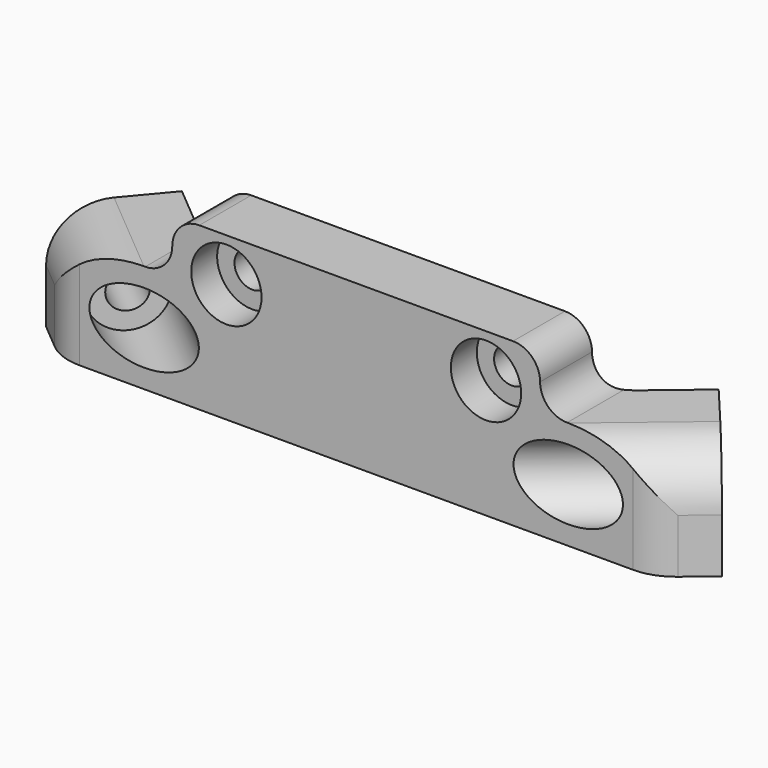
from build123d import *

# Parameters (mm, degrees)
F1_DEPTH       = 10
F2_W           = 34
F2_H           = 6
F3_DEPTH       = 5
F5_R           = 2.49999
F6_D           = 3.3
F6_CBORE_D     = 6.5
F6_CBORE_DEPTH = 3
F7_T1_DEPTH    = 28.1801488287
F7_T3_DEPTH    = 28.1801488287
F8_R           = 1.65
F9_DEPTH       = 49.9246466694
F10_R          = 1.65
F11_DEPTH      = 49.9246466694
F13_R          = 3.25
F14_DEPTH      = 25
F16_R          = 3.25
F17_DEPTH      = 25


# Not quite as in the source:
# - a fillet or chamfer that OpenCascade refuses, or shapes differently, is made with other operations: its cross-section is extruded or revolved along the edge and cut away or added
# - a fillet or chamfer is up to 0.001 mm smaller than in the source, because OpenCascade refuses the exact size


with BuildPart() as f1:
    # F0 (on Top) → F1 (new body)
    with BuildSketch(Plane.XY):
        with BuildLine():
            Line((-25.5868655417, 0), (0, 0))
            Line((0, 0), (25.5868655417, 0))
            ThreePointArc((25.5868655417, 0), (27.2969662583, 0.3015368961), (28.8008035901, 1.1697777844))
            Line((28.8008035901, 1.1697777844), (31.2369389286, 3.2139380484))
            Line((31.2369389286, 3.2139380484), (24.8090628318, 10.8743824796))
            Line((24.8090628318, 10.8743824796), (20.3940868771, 7.1697777844))
            ThreePointArc((20.3940868771, 7.1697777844), (18.8902495453, 6.3015368961), (17.1801488287, 6))
            Line((17.1801488287, 6), (0, 6))
            Line((0, 6), (-17.1801488287, 6))
            ThreePointArc((-17.1801488287, 6), (-18.8902495453, 6.3015368961), (-20.3940868771, 7.1697777844))
            Line((-20.3940868771, 7.1697777844), (-24.8090628318, 10.8743824796))
            Line((-24.8090628318, 10.8743824796), (-31.2369389286, 3.2139380484))
            Line((-31.2369389286, 3.2139380484), (-28.8008035901, 1.1697777844))
            ThreePointArc((-28.8008035901, 1.1697777844), (-27.2969662583, 0.3015368961), (-25.5868655417, 0))
        make_face()
    extrude(amount=F1_DEPTH)

    # F2 (on face) → F3 (join)
    with BuildSketch(Plane.XY.offset(10)):
        with Locations((0, 3)):
            Rectangle(F2_W, F2_H)
    extrude(amount=F3_DEPTH)

    # F5 (radius 2.5 in the source; OpenCascade refuses exactly that, so slightly less here)
    f5_edges = [f1.edges().sort_by_distance(p)[0] for p in [
        (17, 3, 10),
        (17, 3, 15),
        (-17, 3, 15),
        (-17, 3, 10),
    ]]
    fillet(f5_edges, radius=F5_R)

    # F6 (through all)
    with Locations(Plane.XZ):
        with Locations((-12, 11), (12, 11)):
            CounterBoreHole(F6_D / 2, F6_CBORE_D / 2, F6_CBORE_DEPTH)

    # F7: fillet of radius 5 on 2 edges, made by hand

    # F7_s2 → F7_t1 (cut)
    with BuildSketch(Plane(origin=(-29.4886993176, 24.7439567213, 0), x_dir=(0, 0, 1), z_dir=(0.7660444431, -0.6427876097, 0))):
        with BuildLine():
            ThreePointArc((10, 12.6166979253), (8.5355339059, 16.1522318313), (5, 17.6166979253))
            Line((5, 17.6166979253), (10, 17.6166979253))
            Line((10, 17.6166979253), (10, 12.6166979253))
        make_face()
    extrude(amount=F7_T1_DEPTH, mode=Mode.SUBTRACT)

    # F7_s4 → F7_t3 (cut)
    with BuildSketch(Plane(origin=(7.9014529012, 6.6301062151, 0), x_dir=(0, 0, 1), z_dir=(0.7660444431, 0.6427876097, 0))):
        with BuildLine():
            ThreePointArc((5, 17.6166979253), (8.5355339059, 16.1522318313), (10, 12.6166979253))
            Line((10, 12.6166979253), (10, 17.6166979253))
            Line((10, 17.6166979253), (5, 17.6166979253))
        make_face()
    extrude(amount=F7_T3_DEPTH, mode=Mode.SUBTRACT)

    # F8 (on face) → F9 (cut, through all)
    with BuildSketch(Plane(origin=(19.9131437786, 16.7091116002, 0), x_dir=(-0.6427876097, 0.7660444431, 0), z_dir=(0.7660444431, 0.6427876097, 0))):
        with Locations((-12.6166979253, 5)):
            Circle(F8_R)
    extrude(amount=-F9_DEPTH, mode=Mode.SUBTRACT)

    # F10 (on face) → F11 (cut, through all)
    with BuildSketch(Plane(origin=(-19.9131437786, 16.7091116002, 0), x_dir=(-0.6427876097, -0.7660444431, 0), z_dir=(-0.7660444431, 0.6427876097, 0))):
        with Locations((12.6166979253, 5)):
            Circle(F10_R)
    extrude(amount=-F11_DEPTH, mode=Mode.SUBTRACT)

    # F13 (on offset) → F14 (cut)
    with BuildSketch(Plane(origin=(16.082921563, 13.4951735518, 0), x_dir=(-0.6427876097, 0.7660444431, 0), z_dir=(0.7660444431, 0.6427876097, 0))):
        with Locations((-12.6, 5)):
            Circle(F13_R)
    extrude(amount=-F14_DEPTH, mode=Mode.SUBTRACT)

    # F16 (on offset) → F17 (cut)
    with BuildSketch(Plane(origin=(-16.082921563, 13.4951735518, 0), x_dir=(-0.6427876097, -0.7660444431, 0), z_dir=(-0.7660444431, 0.6427876097, 0))):
        with Locations((12.6, 5)):
            Circle(F16_R)
    extrude(amount=-F17_DEPTH, mode=Mode.SUBTRACT)


solid = f1.part
